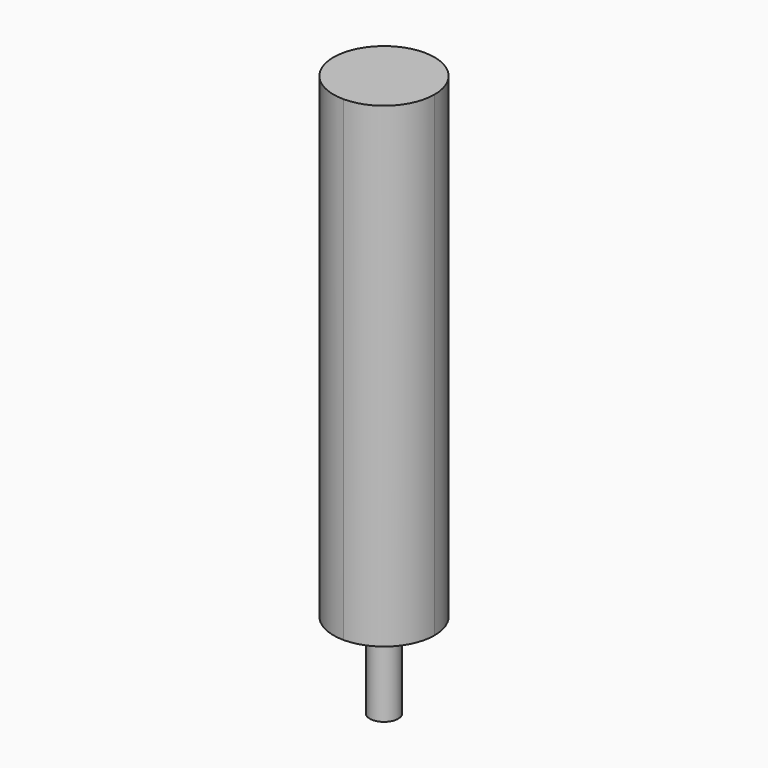
from build123d import *

# Parameters (mm, degrees)
F0_W        = 17.78
F0_H        = 17.78
F1_DEPTH    = 83.82
F2_R        = 2.5
F3_DEPTH    = 15
F4_R        = 2
F5_DEPTH    = 6.35
F6_T1_DEPTH = 128.27


# Not quite as in the source:
# - a fillet or chamfer that OpenCascade refuses, or shapes differently, is made with other operations: its cross-section is extruded or revolved along the edge and cut away or added


with BuildPart() as f1:
    # F0 (on Top) → F1 (new body)
    with BuildSketch(Plane.XY):
        Rectangle(F0_W, F0_H)
    extrude(amount=F1_DEPTH)

    # F2 (on face) → F3 (join)
    with BuildSketch(Plane(origin=(0, 0, 0), x_dir=(1, 0, 0), z_dir=(0, 0, -1))):
        Circle(F2_R)
    extrude(amount=F3_DEPTH)

    # F4 (on face) → F5 (cut)
    with BuildSketch(Plane(origin=(0, 8.89, 0), x_dir=(-1, 0, 0), z_dir=(0, 1, 0))):
        with Locations((0, 3.5875)):
            Circle(F4_R)
        with Locations((0, 80.2325)):
            Circle(F4_R)
    extrude(amount=-F5_DEPTH, mode=Mode.SUBTRACT)

    # F6: fillet of radius 8.89 on 4 edges, made by hand

    # F6_s2 → F6_t1 (cut)
    with BuildSketch(Plane.XY.offset(-22.225)):
        with BuildLine():
            ThreePointArc((8.89, 0), (6.2861792847, -6.2861792847), (0, -8.89))
            Line((0, -8.89), (8.89, -8.89))
            Line((8.89, -8.89), (8.89, 0))
        make_face()
        with BuildLine():
            ThreePointArc((8.89, 0), (6.2861792847, 6.2861792847), (0, 8.89))
            Line((0, 8.89), (8.89, 8.89))
            Line((8.89, 8.89), (8.89, 0))
        make_face()
        with BuildLine():
            ThreePointArc((0, 8.89), (-6.2861792847, 6.2861792847), (-8.89, 0))
            Line((-8.89, 0), (-8.89, 8.89))
            Line((-8.89, 8.89), (0, 8.89))
        make_face()
        with BuildLine():
            ThreePointArc((0, -8.89), (-6.2861792847, -6.2861792847), (-8.89, 0))
            Line((-8.89, 0), (-8.89, -8.89))
            Line((-8.89, -8.89), (0, -8.89))
        make_face()
    extrude(amount=F6_T1_DEPTH, mode=Mode.SUBTRACT)


solid = f1.part
